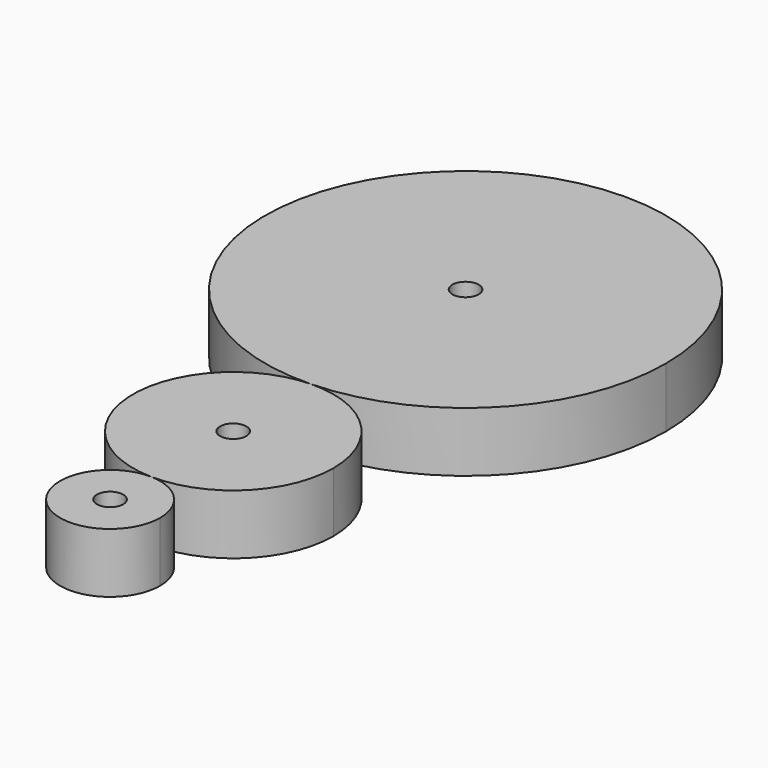
from build123d import *

# Parameters (mm, degrees)
F0_R     = 1.397
F5_DEPTH = 6.35
F6_DEPTH = 6.35
F7_DEPTH = 6.35


# Not quite as in the source:
# - the program builds the solid bodies; features that only make, move or delete a surface that nothing else refers to are left out


with BuildPart() as f5:
    # F0 (on Top) → F5 (new body)
    with BuildSketch(Plane.XY):
        with BuildLine():
            ThreePointArc((-21.2893928371, 25.5092685574), (-6.6169283749, 31.9349210812), (-0.5863672337, 46.7741446483))
            ThreePointArc((-0.5863672337, 46.7741446483), (-37.1008060925, 61.6133682154), (-21.2893928371, 25.5092685574))
        make_face()
        with Locations((-21.8588672337, 46.7741446483)):
            Circle(F0_R, mode=Mode.SUBTRACT)
    extrude(amount=F5_DEPTH)

    # F0 (on Top) → F6 (join)
    with BuildSketch(Plane.XY):
        with BuildLine():
            ThreePointArc((-10.3684056873, 14.8768305106), (-13.5850438864, 22.4977999231), (-21.2893928371, 25.5092685574))
            ThreePointArc((-21.2893928371, 25.5092685574), (-31.640848297, 14.8418900995), (-21.219531291, 4.2427512116))
            ThreePointArc((-21.219531291, 4.2427512116), (-13.5600487997, 7.2802758737), (-10.3684056873, 14.8768305106))
        make_face()
        with Locations((-21.0046556873, 14.8768305106)):
            Circle(F0_R, mode=Mode.SUBTRACT)
    extrude(amount=F6_DEPTH)

    # F0 (on Top) → F7 (join)
    with BuildSketch(Plane.XY):
        with BuildLine():
            ThreePointArc((-16.0206653431, -1.0622259004), (-17.5370650156, 2.6516329184), (-21.219531291, 4.2427512116))
            ThreePointArc((-21.219531291, 4.2427512116), (-25.1163856705, -4.7760847192), (-16.0206653431, -1.0622259004))
        make_face()
        with Locations((-21.3267253431, -1.0622259004)):
            Circle(F0_R, mode=Mode.SUBTRACT)
    extrude(amount=F7_DEPTH)


solid = f5.part
